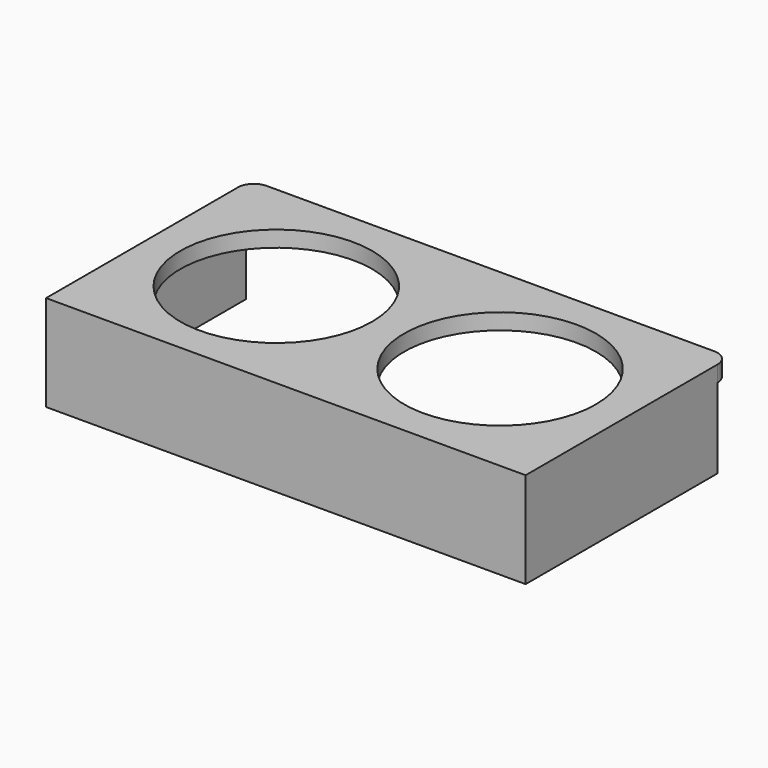
from build123d import *

# Parameters (mm, degrees)
F0_R          = 30
F2_DEPTH      = 5
F1_E0_TOP_W   = 150
F1_E0_TOP_H   = 25
F3_DEPTH      = 2.5
F5_E0_RIGHT_W = 75
F5_E0_RIGHT_H = 25
F6_DEPTH      = 2.5
F4_E0_LEFT_W  = 75
F4_E0_LEFT_H  = 25
F7_DEPTH      = 2.5


with BuildPart() as f2:
    # F0 (on Top) → F2 (new body)
    with BuildSketch(Plane.XY):
        with BuildLine():
            Line((54.8585835038, 26.6114953801), (-85.1414164962, 26.6114953801))
            ThreePointArc((-85.1414164962, 26.6114953801), (-88.6769504021, 25.1470292861), (-90.1414164962, 21.6114953801))
            Line((-90.1414164962, 21.6114953801), (-90.1414164962, -53.3885046199))
            Line((-90.1414164962, -53.3885046199), (59.8585835038, -53.3885046199))
            Line((59.8585835038, -53.3885046199), (59.8585835038, 21.6114953801))
            ThreePointArc((59.8585835038, 21.6114953801), (58.3941174097, 25.1470292861), (54.8585835038, 26.6114953801))
        make_face()
        with Locations((-50.1414164962, -13.3885046199)):
            Circle(F0_R, mode=Mode.SUBTRACT)
        with Locations((19.8585835038, -13.3885046199)):
            Circle(F0_R, mode=Mode.SUBTRACT)
    extrude(amount=F2_DEPTH)

    # F1_E0_top (on explicit) → F3 (join)
    with BuildSketch(Plane(origin=(-90.1414164962, -53.3885046199, 0), x_dir=(1, 0, 0), z_dir=(0, 1, 0))):
        with Locations((75, 12.5)):
            Rectangle(F1_E0_TOP_W, F1_E0_TOP_H)
    extrude(amount=F3_DEPTH)

    # F5_E0_right (on explicit) → F6 (join)
    with BuildSketch(Plane(origin=(59.8585835038, 21.6114953801, 0), x_dir=(0, -1, 0), z_dir=(1, 0, 0))):
        with Locations((37.5, 12.5)):
            Rectangle(F5_E0_RIGHT_W, F5_E0_RIGHT_H)
    extrude(amount=-F6_DEPTH)

    # F4_E0_left (on explicit) → F7 (join)
    with BuildSketch(Plane(origin=(-90.1414164962, 21.6114953801, 0), x_dir=(0, -1, 0), z_dir=(1, 0, 0))):
        with Locations((37.5, 12.5)):
            Rectangle(F4_E0_LEFT_W, F4_E0_LEFT_H)
    extrude(amount=F7_DEPTH)


solid = f2.part
